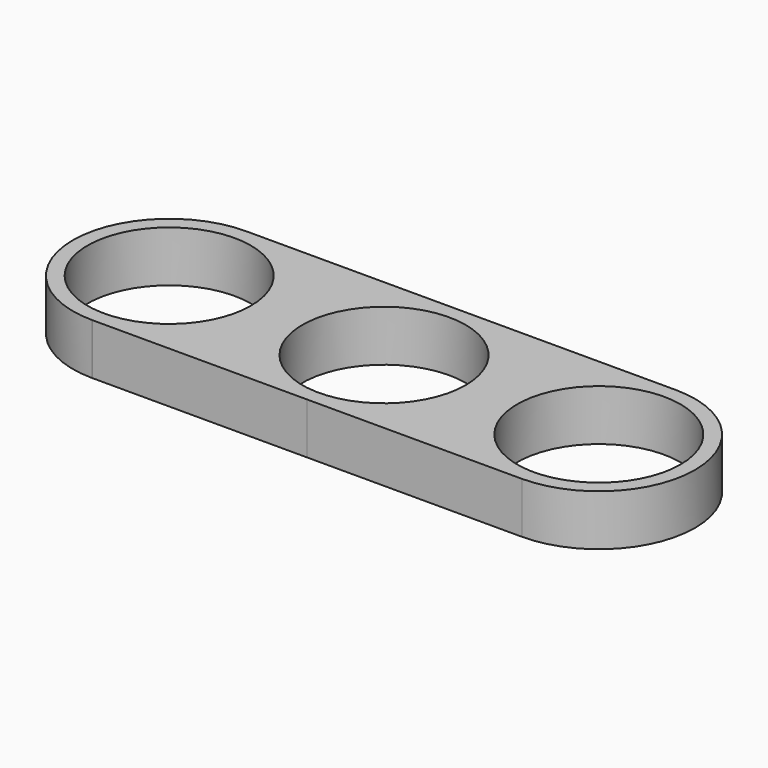
from build123d import *

# Parameters (mm, degrees)
F0_R     = 11.2
F1_DEPTH = 7


# Not quite as in the source:
# - ends of sketch curves that miss each other by under 0.0002 mm in the source are joined


with BuildPart() as f1:
    # F0 (on Top) → F1 (new body)
    with BuildSketch(Plane.XY):
        with BuildLine():
            ThreePointArc((-8.6004e-06, -13.2), (-13.2, 0), (-8.6004e-06, 13.2))
            Line((-8.6004e-06, 13.2), (-29.4360226951, 13.1999579737))
            ThreePointArc((-29.4360226951, 13.1999579737), (-42.6692934144, 0.0318031051), (-29.4996289049, -13.1999652303))
            ThreePointArc((-29.4996289049, -13.1999652303), (-29.4693403268, -13.2), (-29.4390517487, -13.1999652698))
            Line((-29.4390517487, -13.1999652698), (-8.6004e-06, -13.2))
        make_face()
        with Locations((-29.4693317264, 0)):
            Circle(F0_R, mode=Mode.SUBTRACT)
        with BuildLine():
            ThreePointArc((-8.6004e-06, 13.2), (9.333806471, 9.3338125524), (13.2, 0))
            ThreePointArc((13.2, 0), (9.333806471, -9.3338125524), (-8.6004e-06, -13.2))
            Line((-8.6004e-06, -13.2), (29.4658418158, -13.200003649))
            ThreePointArc((29.4658418158, -13.200003649), (42.6658504162, -3.649e-06), (29.4658418158, 13.199996351))
            Line((29.4658418158, 13.199996351), (-8.6004e-06, 13.2))
        make_face()
        with Locations((29.4658504162, -3.649e-06)):
            Circle(F0_R, mode=Mode.SUBTRACT)
        with BuildLine():
            ThreePointArc((-8.6004e-06, -13.2), (9.333806471, -9.3338125524), (13.2, 0))
            ThreePointArc((13.2, 0), (9.333806471, 9.3338125524), (-8.6004e-06, 13.2))
            ThreePointArc((-8.6004e-06, 13.2), (-13.2, 0), (-8.6004e-06, -13.2))
        make_face()
        Circle(F0_R, mode=Mode.SUBTRACT)
    extrude(amount=F1_DEPTH)


solid = f1.part
